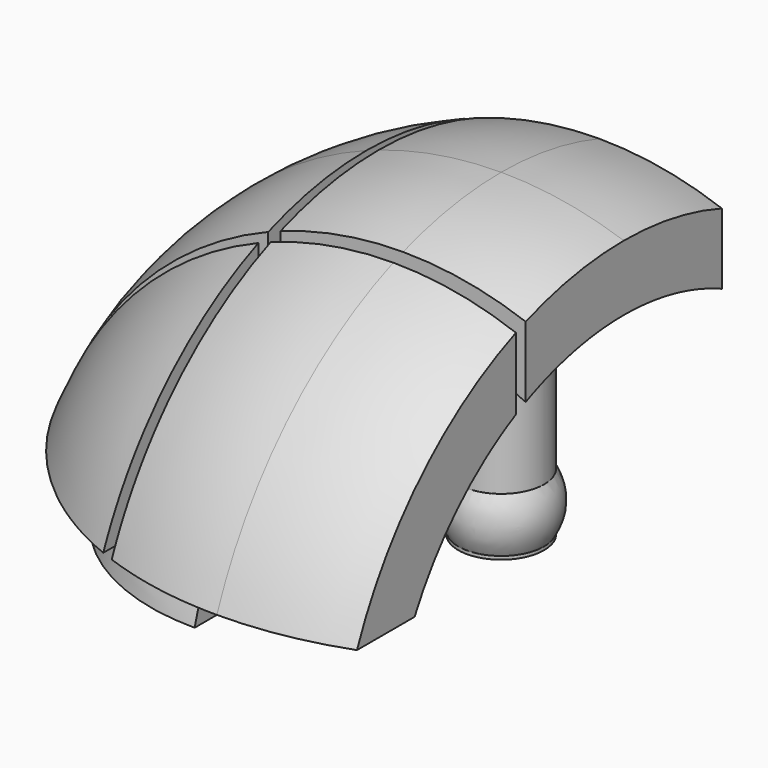
from build123d import *

# Parameters (mm, degrees)
F0_W          = 62
F0_H          = 62
F1_DEPTH      = 31
F2_R          = 30.99999
F3_DEPTH      = 31
F3_DEPTH_BACK = 11
F7_W          = 63
F7_H          = 63
F8_DEPTH      = 18.9837565917
F10_W         = 63
F10_H         = 63
F11_DEPTH     = 1
F13_W         = 63
F13_H         = 63
F14_DEPTH     = 1
F16_W         = 63
F16_H         = 63
F17_DEPTH     = 25
F20_R         = 3.5
F22_DEPTH     = 22
F24_DEPTH     = 25
F28_ANGLE     = 90
F29_ANGLE     = 90


# Not quite as in the source:
# - a fillet or chamfer is up to 0.001 mm smaller than in the source, because OpenCascade refuses the exact size


with BuildPart() as f1:
    # F0 (on Top) → F1 (new body, symmetric)
    with BuildSketch(Plane.XY):
        Rectangle(F0_W, F0_H)
    extrude(amount=F1_DEPTH, both=True)

    # F2 (radius 31 in the source; OpenCascade refuses exactly that, so slightly less here)
    f2_edges = [f1.edges().sort_by_distance(p)[0] for p in [
        (0, 31, 31),
        (-31, 0, 31),
        (0, -31, 31),
        (31, 0, 31),
        (0, 31, -31),
        (-31, 0, -31),
        (0, -31, -31),
        (31, 0, -31),
        (-31, 31, 0),
        (-31, -31, 0),
        (31, -31, 0),
        (31, 31, 0),
    ]]
    fillet(f2_edges, radius=F2_R)

    # F0 (on Top) → F3 (cut, two sides)
    with BuildSketch(Plane.XY) as f3_sk:
        Rectangle(F0_W, F0_H)
    extrude(amount=-F3_DEPTH, mode=Mode.SUBTRACT)
    extrude(f3_sk.sketch, amount=F3_DEPTH_BACK, mode=Mode.SUBTRACT)

    # F4 (on Front) → F5 (revolve, cut)
    with BuildSketch(Plane.XZ):
        with BuildLine():
            Line((0, 26), (0, -26))
            ThreePointArc((0, -26), (26, 0), (0, 26))
        make_face()
    revolve(axis=Axis((0, 0, 0), (0, 0, -1)), mode=Mode.SUBTRACT)

    # F7 (on offset) → F8 (cut, through all)
    with BuildSketch(Plane.YZ.offset(10)):
        Rectangle(F7_W, F7_H)
    extrude(amount=F8_DEPTH, mode=Mode.SUBTRACT)

    # F10 (on offset) → F11 (cut)
    with BuildSketch(Plane.YZ.offset(-10)):
        Rectangle(F10_W, F10_H)
    extrude(amount=-F11_DEPTH, mode=Mode.SUBTRACT)

    # F13 (on offset) → F14 (cut)
    with BuildSketch(Plane.XZ.offset(10)):
        Rectangle(F13_W, F13_H)
    extrude(amount=F14_DEPTH, mode=Mode.SUBTRACT)

    # F16 (on offset) → F17 (cut)
    with BuildSketch(Plane.XZ.offset(-10)):
        with Locations((0, 6.4033556429)):
            Rectangle(F16_W, F16_H)
    extrude(amount=-F17_DEPTH, mode=Mode.SUBTRACT)

    # F20 (on offset) → F22 (join)
    with BuildSketch(Plane.XY.offset(5)):
        Circle(F20_R)
    extrude(amount=F22_DEPTH)

    # F21 (on offset) → F23 (revolve)
    with BuildSketch(Plane.XY.offset(7.5)):
        with BuildLine():
            Line((3.7268394552, -1.8256964905), (-3.7268394552, 1.8256964905))
            ThreePointArc((-3.7268394552, 1.8256964905), (-1.8256964905, -3.7268394552), (3.7268394552, -1.8256964905))
        make_face()
    revolve(axis=Axis((0, 0, 7.5), (0.8980336037, -0.4399268652, 0)))

    # F20 (on offset) → F24 (cut)
    with BuildSketch(Plane.XY.offset(5)):
        Circle(F20_R)
    extrude(amount=-F24_DEPTH, mode=Mode.SUBTRACT)



with BuildPart() as f28:
    # F26 (on offset) → F28 (revolve)
    with BuildSketch(Plane.XZ.offset(6)):
        with BuildLine():
            Line((-11, 11), (-11, 21.3307290077))
            ThreePointArc((-11, 21.3307290077), (-16.9705627485, 16.9705627485), (-21.3307290077, 11))
            Line((-21.3307290077, 11), (-11, 11))
        make_face()
    revolve(axis=Axis((-11, -6, 0), (0, 0, 1)), revolution_arc=F28_ANGLE)


with BuildPart() as f1_1:
    add(f1.part)

    add(f28.part)  # F29 merges F28
    # F27 (on offset) → F29 (revolve)
    with BuildSketch(Plane.XZ.offset(6)):
        with BuildLine():
            Line((-6, 6), (-6, 23.7539470404))
            ThreePointArc((-6, 23.7539470404), (-17.3241161391, 17.3241161391), (-23.7539470404, 6))
            Line((-23.7539470404, 6), (-6, 6))
        make_face()
    revolve(axis=Axis((-6, -6, 14.8769735202), (0, 0, 1)), revolution_arc=F29_ANGLE)


solid = f1_1.part
